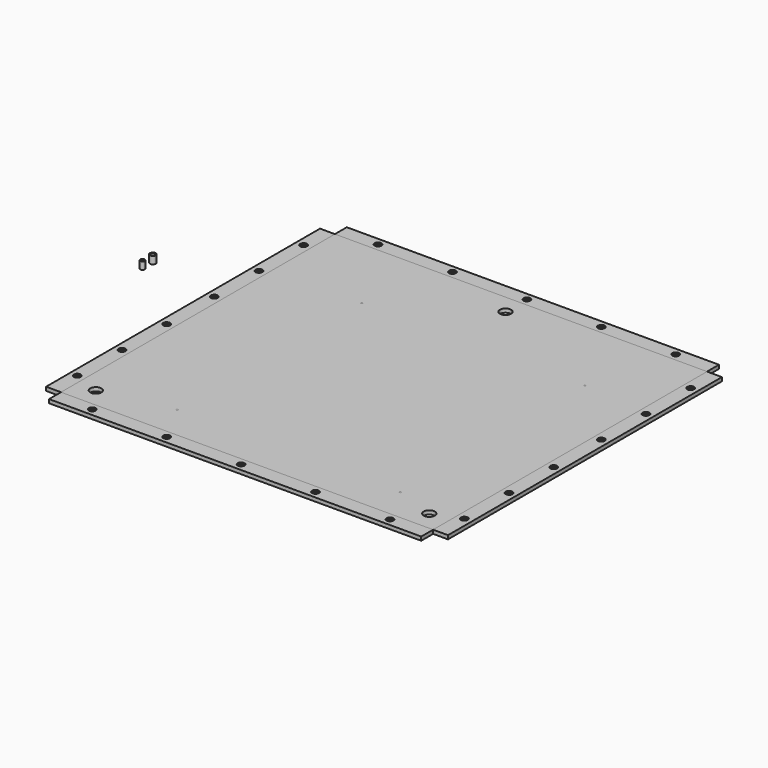
from build123d import *

# Parameters (mm, degrees)
F0_R      = 1.6
F0_R_2    = 2.6
F0_R_3    = 7.5
F0_R_4    = 1.25
F2_DEPTH  = 5
F3_R      = 2.75
F3_R_2    = 1.6
F3_R_3    = 4.6
F3_R_4    = 2.6
F4_DEPTH  = 1.5
F3_R_5    = 11
F3_R_6    = 7.5
F5_DEPTH  = 2
F6_R      = 3
F6_R_2    = 1.6
F7_DEPTH  = 5
F6_R_3    = 4
F6_R_4    = 2.6
F8_DEPTH  = 10
F10_W     = 500
F10_H     = 460
F10_R     = 7.5
F10_R_2   = 1.25
F10_W_2   = 65
F10_H_2   = 280
F11_DEPTH = 5
F12_DEPTH = 3


with BuildPart() as f2:
    # F0 (on Top) → F2 (new body)
    with BuildSketch(Plane.XY):
        Polygon((12.6355909109, 329.2870461196), (-237.3644090891, 329.2870461196), (-237.3644090891, 309.2870461196), (-257.3644090891, 309.2870461196), (-257.3644090891, -150.7129538804), (-237.3644090891, -150.7129538804), (-237.3644090891, -170.7129538804), (262.6355909109, -170.7129538804), (262.6355909109, -150.7129538804), (282.6355909109, -150.7129538804), (282.6355909109, 79.2870461196), (282.6355909109, 309.2870461196), (262.6355909109, 309.2870461196), (262.6355909109, 329.2870461196), align=None)
        with Locations((-226.8644090891, -140.2129538804)):
            Circle(F0_R, mode=Mode.SUBTRACT)
        with Locations((-195.8644090891, -140.2129538804)):
            Circle(F0_R, mode=Mode.SUBTRACT)
        with Locations((-247.3644090891, -110.7129538804)):
            Circle(F0_R_2, mode=Mode.SUBTRACT)
        with Locations((-226.8644090891, -109.2129538804)):
            Circle(F0_R, mode=Mode.SUBTRACT)
        with Locations((-211.3644090891, -124.7129538804)):
            Circle(F0_R_3, mode=Mode.SUBTRACT)
        with Locations((-195.8644090891, -109.2129538804)):
            Circle(F0_R, mode=Mode.SUBTRACT)
        with Locations((-187.3644090891, -160.7129538804)):
            Circle(F0_R_2, mode=Mode.SUBTRACT)
        with Locations((-204.3644090891, -70.8129538804)):
            Circle(F0_R_4, mode=Mode.SUBTRACT)
        with Locations((-156.6644090891, -77.1629538804)):
            Circle(F0_R_4, mode=Mode.SUBTRACT)
        with Locations((-87.3644090891, -160.7129538804)):
            Circle(F0_R_2, mode=Mode.SUBTRACT)
        with Locations((-247.3644090891, -35.7129538804)):
            Circle(F0_R_2, mode=Mode.SUBTRACT)
        with Locations((-204.3644090891, 4.1370461196)):
            Circle(F0_R_4, mode=Mode.SUBTRACT)
        with Locations((-156.6644090891, 5.3870461196)):
            Circle(F0_R_4, mode=Mode.SUBTRACT)
        with Locations((-247.3644090891, 39.2870461196)):
            Circle(F0_R_2, mode=Mode.SUBTRACT)
        with Locations((12.6355909109, -160.7129538804)):
            Circle(F0_R_2, mode=Mode.SUBTRACT)
        with Locations((112.6355909109, -160.7129538804)):
            Circle(F0_R_2, mode=Mode.SUBTRACT)
        with Locations((212.6355909109, -160.7129538804)):
            Circle(F0_R_2, mode=Mode.SUBTRACT)
        with Locations((221.1355909109, -140.2129538804)):
            Circle(F0_R, mode=Mode.SUBTRACT)
        with Locations((252.1355909109, -140.2129538804)):
            Circle(F0_R, mode=Mode.SUBTRACT)
        with Locations((236.6355909109, -124.7129538804)):
            Circle(F0_R_3, mode=Mode.SUBTRACT)
        with Locations((221.1355909109, -109.2129538804)):
            Circle(F0_R, mode=Mode.SUBTRACT)
        with Locations((252.1355909109, -109.2129538804)):
            Circle(F0_R, mode=Mode.SUBTRACT)
        with Locations((272.6355909109, -110.7129538804)):
            Circle(F0_R_2, mode=Mode.SUBTRACT)
        with Locations((272.6355909109, -35.7129538804)):
            Circle(F0_R_2, mode=Mode.SUBTRACT)
        with Locations((272.6355909109, 39.2870461196)):
            Circle(F0_R_2, mode=Mode.SUBTRACT)
        with Locations((-247.3644090891, 119.2870461196)):
            Circle(F0_R_2, mode=Mode.SUBTRACT)
        with Locations((-202.8644090891, 126.7870461196)):
            Circle(F0_R, mode=Mode.SUBTRACT)
        with Locations((-152.8644090891, 126.7870461196)):
            Circle(F0_R, mode=Mode.SUBTRACT)
        with Locations((-247.3644090891, 194.2870461196)):
            Circle(F0_R_2, mode=Mode.SUBTRACT)
        with Locations((-247.3644090891, 269.2870461196)):
            Circle(F0_R_2, mode=Mode.SUBTRACT)
        with Locations((-202.8644090891, 276.7870461196)):
            Circle(F0_R, mode=Mode.SUBTRACT)
        with Locations((-152.8644090891, 276.7870461196)):
            Circle(F0_R, mode=Mode.SUBTRACT)
        with Locations((-187.3644090891, 319.2870461196)):
            Circle(F0_R_2, mode=Mode.SUBTRACT)
        with Locations((-106.8644090891, 267.7870461196)):
            Circle(F0_R, mode=Mode.SUBTRACT)
        with Locations((-91.3644090891, 283.2870461196)):
            Circle(F0_R_3, mode=Mode.SUBTRACT)
        with Locations((-75.8644090891, 267.7870461196)):
            Circle(F0_R, mode=Mode.SUBTRACT)
        with Locations((-106.8644090891, 298.7870461196)):
            Circle(F0_R, mode=Mode.SUBTRACT)
        with Locations((-75.8644090891, 298.7870461196)):
            Circle(F0_R, mode=Mode.SUBTRACT)
        with Locations((-87.3644090891, 319.2870461196)):
            Circle(F0_R_2, mode=Mode.SUBTRACT)
        with Locations((-2.8644090891, 267.7870461196)):
            Circle(F0_R, mode=Mode.SUBTRACT)
        with Locations((-2.8644090891, 298.7870461196)):
            Circle(F0_R, mode=Mode.SUBTRACT)
        with Locations((272.6355909109, 119.2870461196)):
            Circle(F0_R_2, mode=Mode.SUBTRACT)
        with Locations((272.6355909109, 194.2870461196)):
            Circle(F0_R_2, mode=Mode.SUBTRACT)
        with Locations((28.1355909109, 267.7870461196)):
            Circle(F0_R, mode=Mode.SUBTRACT)
        with Locations((12.6355909109, 283.2870461196)):
            Circle(F0_R_3, mode=Mode.SUBTRACT)
        with Locations((28.1355909109, 298.7870461196)):
            Circle(F0_R, mode=Mode.SUBTRACT)
        with Locations((12.6355909109, 319.2870461196)):
            Circle(F0_R_2, mode=Mode.SUBTRACT)
        with Locations((101.1355909109, 267.7870461196)):
            Circle(F0_R, mode=Mode.SUBTRACT)
        with Locations((132.1355909109, 267.7870461196)):
            Circle(F0_R, mode=Mode.SUBTRACT)
        with Locations((116.6355909109, 283.2870461196)):
            Circle(F0_R_3, mode=Mode.SUBTRACT)
        with Locations((101.1355909109, 298.7870461196)):
            Circle(F0_R, mode=Mode.SUBTRACT)
        with Locations((112.6355909109, 319.2870461196)):
            Circle(F0_R_2, mode=Mode.SUBTRACT)
        with Locations((132.1355909109, 298.7870461196)):
            Circle(F0_R, mode=Mode.SUBTRACT)
        with Locations((212.6355909109, 319.2870461196)):
            Circle(F0_R_2, mode=Mode.SUBTRACT)
        with Locations((272.6355909109, 269.2870461196)):
            Circle(F0_R_2, mode=Mode.SUBTRACT)
    extrude(amount=F2_DEPTH)

    # F3 (on face) → F4 (cut)
    with BuildSketch(Plane.XY.offset(5)):
        with Locations((-202.8644090891, 276.7870461196)):
            Circle(F3_R)
        with Locations((-202.8644090891, 276.7870461196)):
            Circle(F3_R_2, mode=Mode.SUBTRACT)
        with Locations((-152.8644090891, 276.7870461196)):
            Circle(F3_R)
        with Locations((-152.8644090891, 276.7870461196)):
            Circle(F3_R_2, mode=Mode.SUBTRACT)
        with Locations((-106.8644090891, 267.7870461196)):
            Circle(F3_R)
        with Locations((-106.8644090891, 267.7870461196)):
            Circle(F3_R_2, mode=Mode.SUBTRACT)
        with Locations((272.6355909109, 269.2870461196)):
            Circle(F3_R_3)
        with Locations((272.6355909109, 269.2870461196)):
            Circle(F3_R_4, mode=Mode.SUBTRACT)
        with Locations((-106.8644090891, 298.7870461196)):
            Circle(F3_R)
        with Locations((-106.8644090891, 298.7870461196)):
            Circle(F3_R_2, mode=Mode.SUBTRACT)
        with Locations((-75.8644090891, 298.7870461196)):
            Circle(F3_R)
        with Locations((-75.8644090891, 298.7870461196)):
            Circle(F3_R_2, mode=Mode.SUBTRACT)
        with Locations((-75.8644090891, 267.7870461196)):
            Circle(F3_R)
        with Locations((-75.8644090891, 267.7870461196)):
            Circle(F3_R_2, mode=Mode.SUBTRACT)
        with Locations((101.1355909109, 298.7870461196)):
            Circle(F3_R)
        with Locations((101.1355909109, 298.7870461196)):
            Circle(F3_R_2, mode=Mode.SUBTRACT)
        with Locations((101.1355909109, 267.7870461196)):
            Circle(F3_R)
        with Locations((101.1355909109, 267.7870461196)):
            Circle(F3_R_2, mode=Mode.SUBTRACT)
        with Locations((132.1355909109, 298.7870461196)):
            Circle(F3_R)
        with Locations((132.1355909109, 298.7870461196)):
            Circle(F3_R_2, mode=Mode.SUBTRACT)
        with Locations((-202.8644090891, 126.7870461196)):
            Circle(F3_R)
        with Locations((-202.8644090891, 126.7870461196)):
            Circle(F3_R_2, mode=Mode.SUBTRACT)
        with Locations((-152.8644090891, 126.7870461196)):
            Circle(F3_R)
        with Locations((-152.8644090891, 126.7870461196)):
            Circle(F3_R_2, mode=Mode.SUBTRACT)
        with Locations((-187.3644090891, -160.7129538804)):
            Circle(F3_R_3)
        with Locations((-187.3644090891, -160.7129538804)):
            Circle(F3_R_4, mode=Mode.SUBTRACT)
        with Locations((-87.3644090891, -160.7129538804)):
            Circle(F3_R_3)
        with Locations((-87.3644090891, -160.7129538804)):
            Circle(F3_R_4, mode=Mode.SUBTRACT)
        with Locations((12.6355909109, -160.7129538804)):
            Circle(F3_R_3)
        with Locations((12.6355909109, -160.7129538804)):
            Circle(F3_R_4, mode=Mode.SUBTRACT)
        with Locations((112.6355909109, -160.7129538804)):
            Circle(F3_R_3)
        with Locations((112.6355909109, -160.7129538804)):
            Circle(F3_R_4, mode=Mode.SUBTRACT)
        with Locations((-195.8644090891, -109.2129538804)):
            Circle(F3_R)
        with Locations((-195.8644090891, -109.2129538804)):
            Circle(F3_R_2, mode=Mode.SUBTRACT)
        with Locations((-226.8644090891, -109.2129538804)):
            Circle(F3_R)
        with Locations((-226.8644090891, -109.2129538804)):
            Circle(F3_R_2, mode=Mode.SUBTRACT)
        with Locations((-226.8644090891, -140.2129538804)):
            Circle(F3_R)
        with Locations((-226.8644090891, -140.2129538804)):
            Circle(F3_R_2, mode=Mode.SUBTRACT)
        with Locations((-195.8644090891, -140.2129538804)):
            Circle(F3_R)
        with Locations((-195.8644090891, -140.2129538804)):
            Circle(F3_R_2, mode=Mode.SUBTRACT)
        with Locations((272.6355909109, 39.2870461196)):
            Circle(F3_R_3)
        with Locations((272.6355909109, 39.2870461196)):
            Circle(F3_R_4, mode=Mode.SUBTRACT)
        with Locations((272.6355909109, -35.7129538804)):
            Circle(F3_R_3)
        with Locations((272.6355909109, -35.7129538804)):
            Circle(F3_R_4, mode=Mode.SUBTRACT)
        with Locations((272.6355909109, -110.7129538804)):
            Circle(F3_R_3)
        with Locations((272.6355909109, -110.7129538804)):
            Circle(F3_R_4, mode=Mode.SUBTRACT)
        with Locations((221.1355909109, -109.2129538804)):
            Circle(F3_R)
        with Locations((221.1355909109, -109.2129538804)):
            Circle(F3_R_2, mode=Mode.SUBTRACT)
        with Locations((252.1355909109, -140.2129538804)):
            Circle(F3_R)
        with Locations((252.1355909109, -140.2129538804)):
            Circle(F3_R_2, mode=Mode.SUBTRACT)
        with Locations((221.1355909109, -140.2129538804)):
            Circle(F3_R)
        with Locations((221.1355909109, -140.2129538804)):
            Circle(F3_R_2, mode=Mode.SUBTRACT)
        with Locations((252.1355909109, -109.2129538804)):
            Circle(F3_R)
        with Locations((252.1355909109, -109.2129538804)):
            Circle(F3_R_2, mode=Mode.SUBTRACT)
        with Locations((272.6355909109, 119.2870461196)):
            Circle(F3_R_3)
        with Locations((272.6355909109, 119.2870461196)):
            Circle(F3_R_4, mode=Mode.SUBTRACT)
        with Locations((272.6355909109, 194.2870461196)):
            Circle(F3_R_3)
        with Locations((272.6355909109, 194.2870461196)):
            Circle(F3_R_4, mode=Mode.SUBTRACT)
        with Locations((132.1355909109, 267.7870461196)):
            Circle(F3_R)
        with Locations((132.1355909109, 267.7870461196)):
            Circle(F3_R_2, mode=Mode.SUBTRACT)
        with Locations((212.6355909109, -160.7129538804)):
            Circle(F3_R_3)
        with Locations((212.6355909109, -160.7129538804)):
            Circle(F3_R_4, mode=Mode.SUBTRACT)
        with Locations((-2.8644090891, 298.7870461196)):
            Circle(F3_R)
        with Locations((-2.8644090891, 298.7870461196)):
            Circle(F3_R_2, mode=Mode.SUBTRACT)
        with Locations((28.1355909109, 298.7870461196)):
            Circle(F3_R)
        with Locations((28.1355909109, 298.7870461196)):
            Circle(F3_R_2, mode=Mode.SUBTRACT)
        with Locations((28.1355909109, 267.7870461196)):
            Circle(F3_R)
        with Locations((28.1355909109, 267.7870461196)):
            Circle(F3_R_2, mode=Mode.SUBTRACT)
        with Locations((-2.8644090891, 267.7870461196)):
            Circle(F3_R)
        with Locations((-2.8644090891, 267.7870461196)):
            Circle(F3_R_2, mode=Mode.SUBTRACT)
    extrude(amount=-F4_DEPTH, mode=Mode.SUBTRACT)

    # F3 (on face) → F5 (cut)
    with BuildSketch(Plane.XY.offset(5)):
        with Locations((-211.3644090891, -124.7129538804)):
            Circle(F3_R_5)
        with Locations((-211.3644090891, -124.7129538804)):
            Circle(F3_R_6, mode=Mode.SUBTRACT)
        with Locations((236.6355909109, -124.7129538804)):
            Circle(F3_R_5)
        with Locations((236.6355909109, -124.7129538804)):
            Circle(F3_R_6, mode=Mode.SUBTRACT)
        with Locations((116.6355909109, 283.2870461196)):
            Circle(F3_R_5)
        with Locations((116.6355909109, 283.2870461196)):
            Circle(F3_R_6, mode=Mode.SUBTRACT)
        with Locations((-91.3644090891, 283.2870461196)):
            Circle(F3_R_5)
        with Locations((-91.3644090891, 283.2870461196)):
            Circle(F3_R_6, mode=Mode.SUBTRACT)
        with Locations((12.6355909109, 283.2870461196)):
            Circle(F3_R_5)
        with Locations((12.6355909109, 283.2870461196)):
            Circle(F3_R_6, mode=Mode.SUBTRACT)
        with Locations((-247.3644090891, 269.2870461196)):
            Circle(F3_R_3)
        with Locations((-247.3644090891, 269.2870461196)):
            Circle(F3_R_4, mode=Mode.SUBTRACT)
        with Locations((-187.3644090891, 319.2870461196)):
            Circle(F3_R_3)
        with Locations((-187.3644090891, 319.2870461196)):
            Circle(F3_R_4, mode=Mode.SUBTRACT)
        with Locations((-87.3644090891, 319.2870461196)):
            Circle(F3_R_3)
        with Locations((-87.3644090891, 319.2870461196)):
            Circle(F3_R_4, mode=Mode.SUBTRACT)
        with Locations((12.6355909109, 319.2870461196)):
            Circle(F3_R_3)
        with Locations((12.6355909109, 319.2870461196)):
            Circle(F3_R_4, mode=Mode.SUBTRACT)
        with Locations((112.6355909109, 319.2870461196)):
            Circle(F3_R_3)
        with Locations((112.6355909109, 319.2870461196)):
            Circle(F3_R_4, mode=Mode.SUBTRACT)
        with Locations((212.6355909109, 319.2870461196)):
            Circle(F3_R_3)
        with Locations((212.6355909109, 319.2870461196)):
            Circle(F3_R_4, mode=Mode.SUBTRACT)
        with Locations((272.6355909109, 269.2870461196)):
            Circle(F3_R_3)
        with Locations((272.6355909109, 269.2870461196)):
            Circle(F3_R_4, mode=Mode.SUBTRACT)
        with Locations((-247.3644090891, 194.2870461196)):
            Circle(F3_R_3)
        with Locations((-247.3644090891, 194.2870461196)):
            Circle(F3_R_4, mode=Mode.SUBTRACT)
        with Locations((-247.3644090891, 119.2870461196)):
            Circle(F3_R_3)
        with Locations((-247.3644090891, 119.2870461196)):
            Circle(F3_R_4, mode=Mode.SUBTRACT)
        with Locations((-247.3644090891, 39.2870461196)):
            Circle(F3_R_3)
        with Locations((-247.3644090891, 39.2870461196)):
            Circle(F3_R_4, mode=Mode.SUBTRACT)
        with Locations((-247.3644090891, -35.7129538804)):
            Circle(F3_R_3)
        with Locations((-247.3644090891, -35.7129538804)):
            Circle(F3_R_4, mode=Mode.SUBTRACT)
        with Locations((-247.3644090891, -110.7129538804)):
            Circle(F3_R_3)
        with Locations((-247.3644090891, -110.7129538804)):
            Circle(F3_R_4, mode=Mode.SUBTRACT)
        with Locations((-187.3644090891, -160.7129538804)):
            Circle(F3_R_3)
        with Locations((-187.3644090891, -160.7129538804)):
            Circle(F3_R_4, mode=Mode.SUBTRACT)
        with Locations((-87.3644090891, -160.7129538804)):
            Circle(F3_R_3)
        with Locations((-87.3644090891, -160.7129538804)):
            Circle(F3_R_4, mode=Mode.SUBTRACT)
        with Locations((12.6355909109, -160.7129538804)):
            Circle(F3_R_3)
        with Locations((12.6355909109, -160.7129538804)):
            Circle(F3_R_4, mode=Mode.SUBTRACT)
        with Locations((112.6355909109, -160.7129538804)):
            Circle(F3_R_3)
        with Locations((112.6355909109, -160.7129538804)):
            Circle(F3_R_4, mode=Mode.SUBTRACT)
        with Locations((272.6355909109, 39.2870461196)):
            Circle(F3_R_3)
        with Locations((272.6355909109, 39.2870461196)):
            Circle(F3_R_4, mode=Mode.SUBTRACT)
        with Locations((272.6355909109, -35.7129538804)):
            Circle(F3_R_3)
        with Locations((272.6355909109, -35.7129538804)):
            Circle(F3_R_4, mode=Mode.SUBTRACT)
        with Locations((272.6355909109, -110.7129538804)):
            Circle(F3_R_3)
        with Locations((272.6355909109, -110.7129538804)):
            Circle(F3_R_4, mode=Mode.SUBTRACT)
        with Locations((272.6355909109, 119.2870461196)):
            Circle(F3_R_3)
        with Locations((272.6355909109, 119.2870461196)):
            Circle(F3_R_4, mode=Mode.SUBTRACT)
        with Locations((272.6355909109, 194.2870461196)):
            Circle(F3_R_3)
        with Locations((272.6355909109, 194.2870461196)):
            Circle(F3_R_4, mode=Mode.SUBTRACT)
        with Locations((212.6355909109, -160.7129538804)):
            Circle(F3_R_3)
        with Locations((212.6355909109, -160.7129538804)):
            Circle(F3_R_4, mode=Mode.SUBTRACT)
        with Locations((272.6355909109, -110.7129538804)):
            Circle(F3_R_4)
        with Locations((212.6355909109, -160.7129538804)):
            Circle(F3_R_4)
        with Locations((272.6355909109, -35.7129538804)):
            Circle(F3_R_4)
        with Locations((112.6355909109, -160.7129538804)):
            Circle(F3_R_4)
        with Locations((272.6355909109, 39.2870461196)):
            Circle(F3_R_4)
        with Locations((272.6355909109, 119.2870461196)):
            Circle(F3_R_4)
        with Locations((272.6355909109, 194.2870461196)):
            Circle(F3_R_4)
        with Locations((272.6355909109, 269.2870461196)):
            Circle(F3_R_4)
        with Locations((-187.3644090891, -160.7129538804)):
            Circle(F3_R_4)
        with Locations((-87.3644090891, -160.7129538804)):
            Circle(F3_R_4)
        with Locations((12.6355909109, -160.7129538804)):
            Circle(F3_R_4)
    extrude(amount=-F5_DEPTH, mode=Mode.SUBTRACT)


with BuildPart() as f7:
    # F6 (on Top) → F7 (new body)
    with BuildSketch(Plane.XY):
        with Locations((-351.8798351288, 129.4269926766)):
            Circle(F6_R)
        with Locations((-351.8798351288, 129.4269926766)):
            Circle(F6_R_2, mode=Mode.SUBTRACT)
    extrude(amount=F7_DEPTH)


with BuildPart() as f7b:
    # F6 (on Top) → F7, piece 2 (new body)
    with BuildSketch(Plane.XY):
        with Locations((-351.8798351288, 146.7694063903)):
            Circle(F6_R_3)
        with Locations((-351.8798351288, 146.7694063903)):
            Circle(F6_R_4, mode=Mode.SUBTRACT)
    extrude(amount=F7_DEPTH)


with BuildPart() as f8:
    # F6 (on Top) → F8 (new body)
    with BuildSketch(Plane.XY):
        with Locations((-351.8798351288, 146.7694063903)):
            Circle(F6_R_3)
        with Locations((-351.8798351288, 146.7694063903)):
            Circle(F6_R_4, mode=Mode.SUBTRACT)
    extrude(amount=F8_DEPTH)


with BuildPart() as f8b:
    # F6 (on Top) → F8, piece 2 (new body)
    with BuildSketch(Plane.XY):
        with Locations((-351.8798351288, 129.4269926766)):
            Circle(F6_R)
        with Locations((-351.8798351288, 129.4269926766)):
            Circle(F6_R_2, mode=Mode.SUBTRACT)
    extrude(amount=F8_DEPTH)


with BuildPart() as f11:
    # F10 (on face) → F11 (new body)
    with BuildSketch(Plane.XY):
        with Locations((12.6355909109, 79.2870461196)):
            Rectangle(F10_W, F10_H)
        with Locations((-211.3644090891, -124.7129538804)):
            Circle(F10_R, mode=Mode.SUBTRACT)
        with Locations((236.6355909109, -124.7129538804)):
            Circle(F10_R, mode=Mode.SUBTRACT)
        Polygon((-128.5639107227, -110.7129538804), (-127.3644090891, 209.2870461196), (192.6355909109, 209.2870461196), (192.6355909109, -110.7129538804), (-117.3644090891, -110.7129538804), align=None, mode=Mode.SUBTRACT)
        with Locations((12.6355909109, 283.2870461196)):
            Circle(F10_R, mode=Mode.SUBTRACT)
        Polygon((192.6355909109, 209.2870461196), (-127.3644090891, 209.2870461196), (-128.5639107227, -110.7129538804), (-117.3644090891, -110.7129538804), (192.6355909109, -110.7129538804), align=None)
        with Locations((-117.3644090891, -105.7129538804)):
            Circle(F10_R_2, mode=Mode.SUBTRACT)
        with Locations((-74.8644090891, 49.2870461196)):
            Rectangle(F10_W_2, F10_H_2, mode=Mode.SUBTRACT)
        with Locations((182.6355909109, -105.7129538804)):
            Circle(F10_R_2, mode=Mode.SUBTRACT)
        with Locations((-117.3644090891, 204.2870461196)):
            Circle(F10_R_2, mode=Mode.SUBTRACT)
        with Locations((182.6355909109, 204.2870461196)):
            Circle(F10_R_2, mode=Mode.SUBTRACT)
        with Locations((-74.8644090891, 49.2870461196)):
            Rectangle(F10_W_2, F10_H_2)
    extrude(amount=F11_DEPTH)


with BuildPart() as f12:
    # F10 (on face) → F12 (new body)
    with BuildSketch(Plane.XY):
        Polygon((192.6355909109, 209.2870461196), (-127.3644090891, 209.2870461196), (-128.5639107227, -110.7129538804), (-117.3644090891, -110.7129538804), (192.6355909109, -110.7129538804), align=None)
        with Locations((-117.3644090891, -105.7129538804)):
            Circle(F10_R_2, mode=Mode.SUBTRACT)
        with Locations((-74.8644090891, 49.2870461196)):
            Rectangle(F10_W_2, F10_H_2, mode=Mode.SUBTRACT)
        with Locations((182.6355909109, -105.7129538804)):
            Circle(F10_R_2, mode=Mode.SUBTRACT)
        with Locations((-117.3644090891, 204.2870461196)):
            Circle(F10_R_2, mode=Mode.SUBTRACT)
        with Locations((182.6355909109, 204.2870461196)):
            Circle(F10_R_2, mode=Mode.SUBTRACT)
        with Locations((-74.8644090891, 49.2870461196)):
            Rectangle(F10_W_2, F10_H_2)
    extrude(amount=F12_DEPTH)


solid = Compound([f2.part, f7.part, f7b.part, f8.part, f8b.part, f11.part, f12.part])
